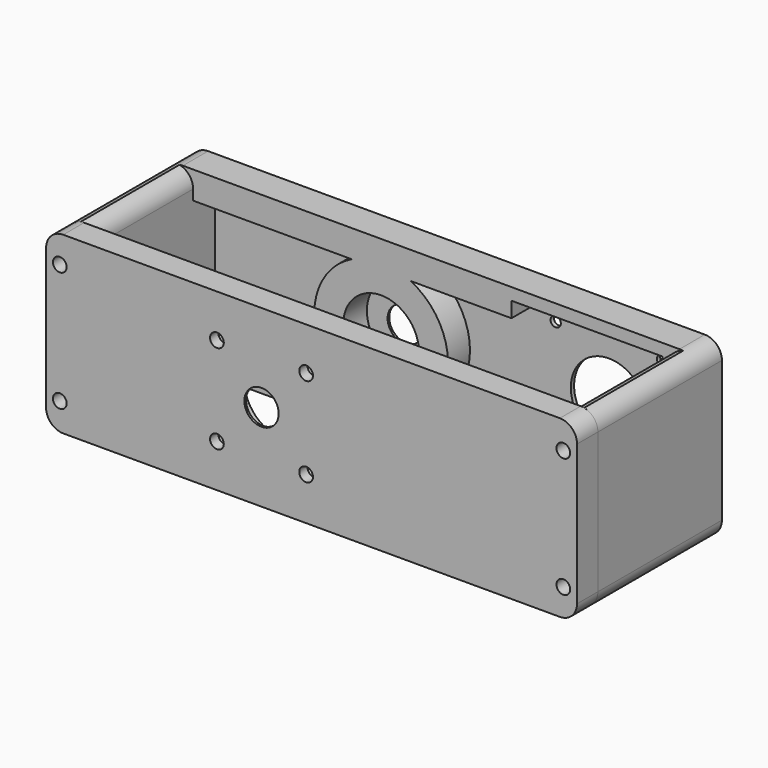
from build123d import *

# Parameters (mm, degrees)
F0_W       = 154.8125
F0_H       = 51
F0_R       = 1.5
F0_R_2     = 11.05
F0_R_3     = 11.1
F1_DEPTH   = 1.2
F2_W       = 154.8125
F2_H       = 51
F2_R       = 11.05
F3_DEPTH   = 8
F4_W       = 8
F4_H       = 51
F5_DEPTH   = 36
F6_W       = 154.8125
F6_H       = 51
F7_DEPTH   = 7.6
F0_R_4     = 5
F8_DEPTH   = 0.6
F9_R       = 11.05
F9_R_2     = 5
F9_R_3     = 2
F10_DEPTH  = 52.801
F11_DEPTH  = 0.6
F14_DEPTH  = 3
F15_R      = 2
F16_DEPTH  = 15
F19_DEPTH  = 3
F20_R      = 2
F21_DEPTH  = 52.801
F22_F1_R   = 5
F22_F2_R   = 5
F22_F3_R   = 5
F22_F4_R   = 5
F22_F5_R   = 5
F22_F6_R   = 5
F22_F7_R   = 5
F22_F8_R   = 5
F22_2_F1_R = 5
F22_2_F2_R = 5
F22_2_F3_R = 5
F22_2_F4_R = 5


with BuildPart() as f1:
    # F0 (on Front) → F1 (new body)
    with BuildSketch(Plane.XZ):
        with Locations((14.59375, 0)):
            Rectangle(F0_W, F0_H)
        with Locations((44.5, -15.5)):
            Circle(F0_R, mode=Mode.SUBTRACT)
        with Locations((75.5, -15.5)):
            Circle(F0_R, mode=Mode.SUBTRACT)
        Circle(F0_R_2, mode=Mode.SUBTRACT)
        with Locations((60, 0)):
            Circle(F0_R_3, mode=Mode.SUBTRACT)
        with Locations((44.5, 15.5)):
            Circle(F0_R, mode=Mode.SUBTRACT)
        with Locations((75.5, 15.5)):
            Circle(F0_R, mode=Mode.SUBTRACT)
    extrude(amount=F1_DEPTH)

    # F2 (on face) → F3 (join)
    with BuildSketch(Plane.XZ.offset(1.2)):
        with Locations((14.59375, 0)):
            Rectangle(F2_W, F2_H)
        with BuildLine():
            Line((-8.602325267, -17.5), (-54.8125, -17.5))
            Line((-54.8125, -17.5), (-54.8125, 17.5))
            Line((-54.8125, 17.5), (-8.602325267, 17.5))
            ThreePointArc((-8.602325267, 17.5), (-19.5, 0), (-8.602325267, -17.5))
        make_face(mode=Mode.SUBTRACT)
        Circle(F2_R, mode=Mode.SUBTRACT)
        with BuildLine():
            Line((82, 17.5), (84, 17.5))
            Line((84, 17.5), (84, -17.5))
            Line((84, -17.5), (82, -17.5))
            Line((82, -17.5), (82, -22))
            Line((82, -22), (38, -22))
            Line((38, -22), (38, -17.5))
            Line((38, -17.5), (8.602325267, -17.5))
            ThreePointArc((8.602325267, -17.5), (19.5, 0), (8.602325267, 17.5))
            Line((8.602325267, 17.5), (38, 17.5))
            Line((38, 17.5), (38, 22))
            Line((38, 22), (82, 22))
            Line((82, 22), (82, 17.5))
        make_face(mode=Mode.SUBTRACT)
    extrude(amount=F3_DEPTH)

    # F4 (on face) → F5 (join)
    with BuildSketch(Plane.XZ.offset(9.2)):
        with Locations((88, 0)):
            Rectangle(F4_W, F4_H)
        with Locations((-58.8125, 0)):
            Rectangle(F4_W, F4_H)
    extrude(amount=F5_DEPTH)

    # F0 (on Front) → F8 (join)
    with BuildSketch(Plane.XZ):
        Circle(F0_R_2)
        Circle(F0_R_4, mode=Mode.SUBTRACT)
    extrude(amount=F8_DEPTH)

    # F15 (on face) → F16 (cut)
    with BuildSketch(Plane.XZ.offset(45.2)):
        with Locations((88, 17.5)):
            Circle(F15_R)
        with Locations((88, -17.5)):
            Circle(F15_R)
        with Locations((-58.8125, 17.5)):
            Circle(F15_R)
        with Locations((-58.8125, -17.5)):
            Circle(F15_R)
    extrude(amount=-F16_DEPTH, mode=Mode.SUBTRACT)

    # F18 (on offset) → F19 (cut)
    with BuildSketch(Plane.XZ.offset(40.2)):
        Polygon((-55.1125, 15.363804004), (-55.1125, 19.636195996), (-58.8125, 21.772391992), (-62.5125, 19.636195996), (-62.5125, 15.363804004), (-58.8125, 13.227608008), align=None)
        Polygon((-55.1125, -19.636195996), (-55.1125, -15.363804004), (-58.8125, -13.227608008), (-62.5125, -15.363804004), (-62.5125, -19.636195996), (-58.8125, -21.772391992), align=None)
        Polygon((84.3, 19.636195996), (84.3, 15.363804004), (88, 13.227608008), (91.7, 15.363804004), (91.7, 19.636195996), (88, 21.772391992), align=None)
        Polygon((84.3, -15.363804004), (84.3, -19.636195996), (88, -21.772391992), (91.7, -19.636195996), (91.7, -15.363804004), (88, -13.227608008), align=None)
    extrude(amount=-F19_DEPTH, mode=Mode.SUBTRACT)

    # F22: fillet of radius 5 on 8 edges, made by hand

    # F22_f1
    f22_f1_edges = [f1.edges().sort_by_distance(p)[0] for p in [
        (84, -27.2, 25.5),
    ]]
    fillet(f22_f1_edges, radius=F22_F1_R)

    # F22_f2
    f22_f2_edges = [f1.edges().sort_by_distance(p)[0] for p in [
        (-54.8125, -27.2, 25.5),
    ]]
    fillet(f22_f2_edges, radius=F22_F2_R)

    # F22_f3
    f22_f3_edges = [f1.edges().sort_by_distance(p)[0] for p in [
        (84, -27.2, -25.5),
    ]]
    fillet(f22_f3_edges, radius=F22_F3_R)

    # F22_f4
    f22_f4_edges = [f1.edges().sort_by_distance(p)[0] for p in [
        (-54.8125, -27.2, -25.5),
    ]]
    fillet(f22_f4_edges, radius=F22_F4_R)

    # F22_f5
    f22_f5_edges = [f1.edges().sort_by_distance(p)[0] for p in [
        (92, -22.6, 25.5),
    ]]
    fillet(f22_f5_edges, radius=F22_F5_R)

    # F22_f6
    f22_f6_edges = [f1.edges().sort_by_distance(p)[0] for p in [
        (-62.8125, -22.6, 25.5),
    ]]
    fillet(f22_f6_edges, radius=F22_F6_R)

    # F22_f7
    f22_f7_edges = [f1.edges().sort_by_distance(p)[0] for p in [
        (92, -22.6, -25.5),
    ]]
    fillet(f22_f7_edges, radius=F22_F7_R)

    # F22_f8
    f22_f8_edges = [f1.edges().sort_by_distance(p)[0] for p in [
        (-62.8125, -22.6, -25.5),
    ]]
    fillet(f22_f8_edges, radius=F22_F8_R)


with BuildPart() as f7:
    # F6 (on face) → F7 (new body)
    with BuildSketch(Plane.XZ.offset(45.2)):
        with Locations((14.59375, 0)):
            Rectangle(F6_W, F6_H)
    extrude(amount=F7_DEPTH)

    # F9 (on face) → F10 (cut, through all)
    with BuildSketch(Plane.XZ.offset(52.8)):
        Circle(F9_R)
        Circle(F9_R_2, mode=Mode.SUBTRACT)
        with Locations((-13, -13)):
            Circle(F9_R_3)
        with Locations((13, -13)):
            Circle(F9_R_3)
        with Locations((13, 13)):
            Circle(F9_R_3)
        with Locations((-13, 13)):
            Circle(F9_R_3)
        Circle(F9_R_2)
    extrude(amount=-F10_DEPTH, mode=Mode.SUBTRACT)

    # F9 (on face) → F11 (join)
    with BuildSketch(Plane.XZ.offset(52.8)):
        Circle(F9_R)
        Circle(F9_R_2, mode=Mode.SUBTRACT)
    extrude(amount=-F11_DEPTH)

    # F13 (on offset) → F14 (cut)
    with BuildSketch(Plane.XZ.offset(49.8)):
        Polygon((-9.3, -15.136195996), (-9.3, -10.863804004), (-13, -8.727608008), (-16.7, -10.863804004), (-16.7, -15.136195996), (-13, -17.272391992), align=None)
        Polygon((-9.3, 10.863804004), (-9.3, 15.136195996), (-13, 17.272391992), (-16.7, 15.136195996), (-16.7, 10.863804004), (-13, 8.727608008), align=None)
        Polygon((9.3, 15.136195996), (9.3, 10.863804004), (13, 8.727608008), (16.7, 10.863804004), (16.7, 15.136195996), (13, 17.272391992), align=None)
        Polygon((9.3, -10.863804004), (9.3, -15.136195996), (13, -17.272391992), (16.7, -15.136195996), (16.7, -10.863804004), (13, -8.727608008), align=None)
    extrude(amount=-F14_DEPTH, mode=Mode.SUBTRACT)

    # F20 (on face) → F21 (cut, through all)
    with BuildSketch(Plane.XZ.offset(52.8)):
        with Locations((-58.8125, -17.5)):
            Circle(F20_R)
        with Locations((-58.8125, 17.5)):
            Circle(F20_R)
        with Locations((88, 17.5)):
            Circle(F20_R)
        with Locations((88, -17.5)):
            Circle(F20_R)
    extrude(amount=-F21_DEPTH, mode=Mode.SUBTRACT)

    # F22#2: fillet of radius 5 on 4 edges, made by hand

    # F22_2_f1
    f22_2_f1_edges = [f7.edges().sort_by_distance(p)[0] for p in [
        (-62.8125, -49, -25.5),
    ]]
    fillet(f22_2_f1_edges, radius=F22_2_F1_R)

    # F22_2_f2
    f22_2_f2_edges = [f7.edges().sort_by_distance(p)[0] for p in [
        (92, -49, -25.5),
    ]]
    fillet(f22_2_f2_edges, radius=F22_2_F2_R)

    # F22_2_f3
    f22_2_f3_edges = [f7.edges().sort_by_distance(p)[0] for p in [
        (-62.8125, -49, 25.5),
    ]]
    fillet(f22_2_f3_edges, radius=F22_2_F3_R)

    # F22_2_f4
    f22_2_f4_edges = [f7.edges().sort_by_distance(p)[0] for p in [
        (92, -49, 25.5),
    ]]
    fillet(f22_2_f4_edges, radius=F22_2_F4_R)


solid = Compound([f1.part, f7.part])
